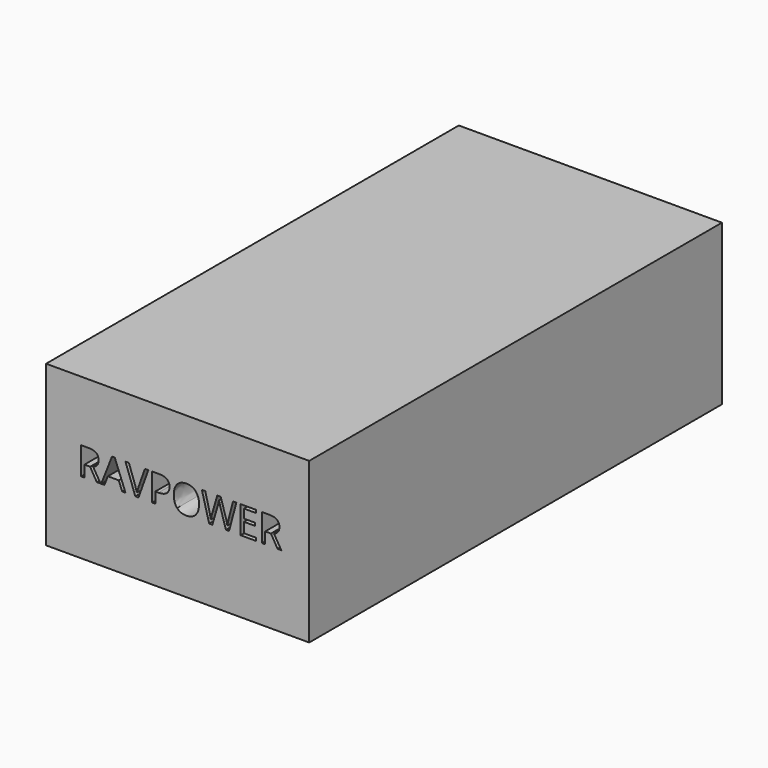
from build123d import *

# Parameters (mm, degrees)
F0_W     = 51
F0_H     = 31
F1_DEPTH = 100


with BuildPart() as f1:
    # F0 (on Front) → F1 (new body)
    with BuildSketch(Plane.XZ):
        with Locations((-41.3011932845, 49.3138737511)):
            Rectangle(F0_W, F0_H)
        with BuildLine():
            Line((-58.2602472687, 50.0083940445), (-59.3696140923, 50.0083940445))
            Line((-59.3696140923, 50.0083940445), (-59.3696140923, 47.7989632636))
            Line((-59.3696140923, 47.7989632636), (-59.9870918526, 47.7989632636))
            Line((-59.9870918526, 47.7989632636), (-59.9870918526, 53.1120628624))
            Line((-59.9870918526, 53.1120628624), (-58.5300303956, 53.1120628624))
            add(Edge.make_bspline(
                [(-58.5300303956, 53.1120628624), (-57.5520665605, 53.1120628624), (-57.0851789507, 52.737622488)],
                knots=[0, 0, 0, 1, 1, 1], degree=2))
            add(Edge.make_bspline(
                [(-57.0851789507, 52.737622488), (-56.618291341, 52.3631821136), (-56.618291341, 51.6108127898)],
                knots=[0, 0, 0, 1, 1, 1], degree=2))
            add(Edge.make_bspline(
                [(-56.618291341, 51.6108127898), (-56.618291341, 50.5572631648), (-57.6869581239, 50.1863113653)],
                knots=[0, 0, 0, 1, 1, 1], degree=2))
            Line((-57.6869581239, 50.1863113653), (-56.2438509665, 47.7989632636))
            Line((-56.2438509665, 47.7989632636), (-56.9741259825, 47.7989632636))
            Line((-56.9741259825, 47.7989632636), (-58.2602472687, 50.0083940445))
        make_face(mode=Mode.SUBTRACT)
        Polygon((-51.4075232731, 47.7989632636), (-52.0470953412, 47.7989632636), (-52.7087617172, 49.4885963818), (-54.8379552749, 49.4885963818), (-55.4914816427, 47.7989632636), (-56.1170994112, 47.7989632636), (-54.0169773111, 53.1341571703), (-53.4971796484, 53.1341571703), align=None, mode=Mode.SUBTRACT)
        with BuildLine():
            Line((-48.8562121503, 49.6955851603), (-47.6421880792, 53.1120628624))
            Line((-47.6421880792, 53.1120628624), (-46.9781959866, 53.1120628624))
            Line((-46.9781959866, 53.1120628624), (-48.8922607578, 47.7989632636))
            Line((-48.8922607578, 47.7989632636), (-49.5027613683, 47.7989632636))
            Line((-49.5027613683, 47.7989632636), (-51.4075232731, 53.1120628624))
            Line((-51.4075232731, 53.1120628624), (-50.752834047, 53.1120628624))
            Line((-50.752834047, 53.1120628624), (-49.531832826, 49.6746537107))
            add(Edge.make_bspline(
                [(-49.531832826, 49.6746537107), (-49.3213554726, 49.0815959748), (-49.1980924922, 48.5222611298)],
                knots=[0, 0, 0, 1, 1, 1], degree=2))
            add(Edge.make_bspline(
                [(-49.1980924922, 48.5222611298), (-49.0666895037, 49.1106674325), (-48.8562121503, 49.6955851603)],
                knots=[0, 0, 0, 1, 1, 1], degree=2))
        make_face(mode=Mode.SUBTRACT)
        with BuildLine():
            add(Edge.make_bspline(
                [(-44.8699338783, 53.1120628624), (-42.879120459, 53.1120628624), (-42.879120459, 51.5642984575)],
                knots=[0, 0, 0, 1, 1, 1], degree=2))
            add(Edge.make_bspline(
                [(-42.879120459, 51.5642984575), (-42.879120459, 50.7572747934), (-43.4297338667, 50.3229472162)],
                knots=[0, 0, 0, 1, 1, 1], degree=2))
            add(Edge.make_bspline(
                [(-43.4297338667, 50.3229472162), (-43.9803472745, 49.888619639), (-45.0048254418, 49.888619639)],
                knots=[0, 0, 0, 1, 1, 1], degree=2))
            Line((-45.0048254418, 49.888619639), (-45.6304432103, 49.888619639))
            Line((-45.6304432103, 49.888619639), (-45.6304432103, 47.7989632636))
            Line((-45.6304432103, 47.7989632636), (-46.2479209706, 47.7989632636))
            Line((-46.2479209706, 47.7989632636), (-46.2479209706, 53.1120628624))
            Line((-46.2479209706, 53.1120628624), (-44.8699338783, 53.1120628624))
        make_face(mode=Mode.SUBTRACT)
        with BuildLine():
            add(Edge.make_bspline(
                [(-37.7985925213, 52.4690022194), (-37.1555318782, 51.7422157783), (-37.1555318782, 50.463071642)],
                knots=[0, 0, 0, 1, 1, 1], degree=2))
            add(Edge.make_bspline(
                [(-37.1555318782, 50.463071642), (-37.1555318782, 49.1874160807), (-37.8009182379, 48.4565596355)],
                knots=[0, 0, 0, 1, 1, 1], degree=2))
            add(Edge.make_bspline(
                [(-37.8009182379, 48.4565596355), (-38.4463045976, 47.7257031904), (-39.5940457453, 47.7257031904)],
                knots=[0, 0, 0, 1, 1, 1], degree=2))
            add(Edge.make_bspline(
                [(-39.5940457453, 47.7257031904), (-40.7673697758, 47.7257031904), (-41.4051975565, 48.4437681942)],
                knots=[0, 0, 0, 1, 1, 1], degree=2))
            add(Edge.make_bspline(
                [(-41.4051975565, 48.4437681942), (-42.0430253371, 49.1618331979), (-42.0430253371, 50.4700487919)],
                knots=[0, 0, 0, 1, 1, 1], degree=2))
            add(Edge.make_bspline(
                [(-42.0430253371, 50.4700487919), (-42.0430253371, 51.767798661), (-41.403453269, 52.4817936607)],
                knots=[0, 0, 0, 1, 1, 1], degree=2))
            add(Edge.make_bspline(
                [(-41.403453269, 52.4817936607), (-40.7638812009, 53.1957886605), (-39.5870685955, 53.1957886605)],
                knots=[0, 0, 0, 1, 1, 1], degree=2))
            add(Edge.make_bspline(
                [(-39.5870685955, 53.1957886605), (-38.4416531643, 53.1957886605), (-37.7985925213, 52.4690022194)],
                knots=[0, 0, 0, 1, 1, 1], degree=2))
        make_face(mode=Mode.SUBTRACT)
        with BuildLine():
            Line((-29.9132503502, 53.1120628624), (-31.3342631998, 47.7989632636))
            Line((-31.3342631998, 47.7989632636), (-31.9447638103, 47.7989632636))
            Line((-31.9447638103, 47.7989632636), (-33.0169191682, 51.3561468208))
            add(Edge.make_bspline(
                [(-33.0169191682, 51.3561468208), (-33.0936678164, 51.5933699152), (-33.1878593391, 51.9526931316)],
                knots=[0, 0, 0, 1, 1, 1], degree=2))
            add(Edge.make_bspline(
                [(-33.1878593391, 51.9526931316), (-33.2820508619, 52.3120163481), (-33.2855394368, 52.3852764214)],
                knots=[0, 0, 0, 1, 1, 1], degree=2))
            add(Edge.make_bspline(
                [(-33.2855394368, 52.3852764214), (-33.3657766599, 51.9050159411), (-33.5402054058, 51.3352153713)],
                knots=[0, 0, 0, 1, 1, 1], degree=2))
            Line((-33.5402054058, 51.3352153713), (-34.5798007311, 47.7989632636))
            Line((-34.5798007311, 47.7989632636), (-35.1903013416, 47.7989632636))
            Line((-35.1903013416, 47.7989632636), (-36.6043370413, 53.1120628624))
            Line((-36.6043370413, 53.1120628624), (-35.9496478152, 53.1120628624))
            Line((-35.9496478152, 53.1120628624), (-35.1100641185, 49.8304767237))
            add(Edge.make_bspline(
                [(-35.1100641185, 49.8304767237), (-34.9356353726, 49.1397388901), (-34.8553981495, 48.5804040451)],
                knots=[0, 0, 0, 1, 1, 1], degree=2))
            add(Edge.make_bspline(
                [(-34.8553981495, 48.5804040451), (-34.7577180518, 49.2455589959), (-34.5646835731, 49.8816424892)],
                knots=[0, 0, 0, 1, 1, 1], degree=2))
            Line((-34.5646835731, 49.8816424892), (-33.613465479, 53.1120628624))
            Line((-33.613465479, 53.1120628624), (-32.9587762529, 53.1120628624))
            Line((-32.9587762529, 53.1120628624), (-31.9598809683, 49.8525710315))
            add(Edge.make_bspline(
                [(-31.9598809683, 49.8525710315), (-31.7854522224, 49.2885847533), (-31.6656778169, 48.5804040451)],
                knots=[0, 0, 0, 1, 1, 1], degree=2))
            add(Edge.make_bspline(
                [(-31.6656778169, 48.5804040451), (-31.5959063186, 49.0967131328), (-31.4040346982, 49.8374538736)],
                knots=[0, 0, 0, 1, 1, 1], degree=2))
            Line((-31.4040346982, 49.8374538736), (-30.5679395763, 53.1120628624))
            Line((-30.5679395763, 53.1120628624), (-29.9132503502, 53.1120628624))
        make_face(mode=Mode.SUBTRACT)
        Polygon((-26.120006557, 48.3513209588), (-26.120006557, 47.7989632636), (-29.0818066616, 47.7989632636), (-29.0818066616, 53.1120628624), (-26.120006557, 53.1120628624), (-26.120006557, 52.5631937421), (-28.4643289013, 52.5631937421), (-28.4643289013, 50.8514663161), (-26.2618752703, 50.8514663161), (-26.2618752703, 50.3060857708), (-28.4643289013, 50.3060857708), (-28.4643289013, 48.3513209588), align=None, mode=Mode.SUBTRACT)
        with BuildLine():
            Line((-23.2163493676, 50.0083940445), (-24.3257161913, 50.0083940445))
            Line((-24.3257161913, 50.0083940445), (-24.3257161913, 47.7989632636))
            Line((-24.3257161913, 47.7989632636), (-24.9431939516, 47.7989632636))
            Line((-24.9431939516, 47.7989632636), (-24.9431939516, 53.1120628624))
            Line((-24.9431939516, 53.1120628624), (-23.4861324945, 53.1120628624))
            add(Edge.make_bspline(
                [(-23.4861324945, 53.1120628624), (-22.5081686594, 53.1120628624), (-22.0412810497, 52.737622488)],
                knots=[0, 0, 0, 1, 1, 1], degree=2))
            add(Edge.make_bspline(
                [(-22.0412810497, 52.737622488), (-21.5743934399, 52.3631821136), (-21.5743934399, 51.6108127898)],
                knots=[0, 0, 0, 1, 1, 1], degree=2))
            add(Edge.make_bspline(
                [(-21.5743934399, 51.6108127898), (-21.5743934399, 50.5572631648), (-22.6430602229, 50.1863113653)],
                knots=[0, 0, 0, 1, 1, 1], degree=2))
            Line((-22.6430602229, 50.1863113653), (-21.1999530655, 47.7989632636))
            Line((-21.1999530655, 47.7989632636), (-21.9302280815, 47.7989632636))
            Line((-21.9302280815, 47.7989632636), (-23.2163493676, 50.0083940445))
        make_face(mode=Mode.SUBTRACT)
    extrude(amount=F1_DEPTH)


solid = f1.part
